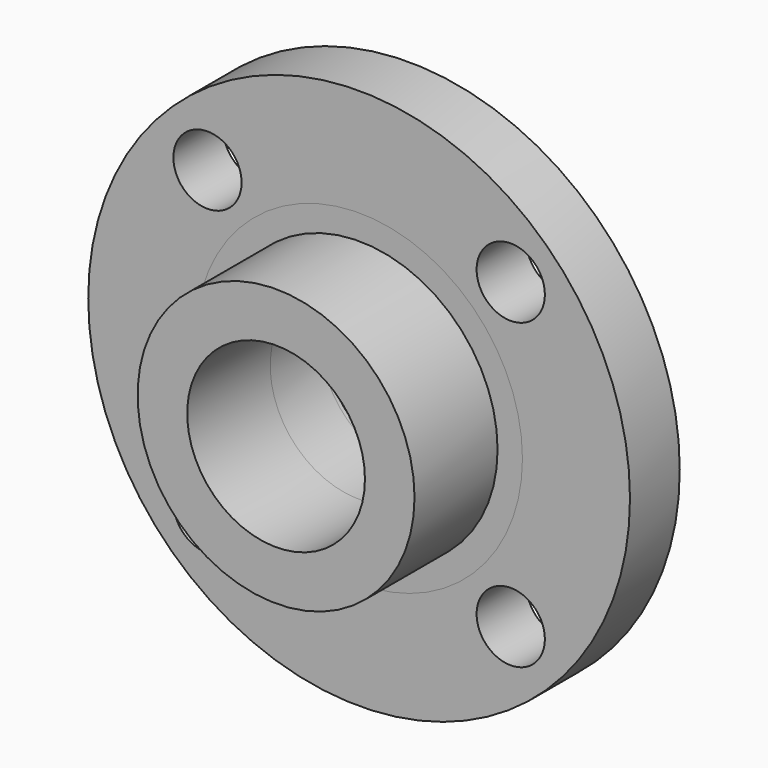
from build123d import *

# Parameters (mm, degrees)
F0_R     = 76.2
F0_R_2   = 9.6012
F0_R_3   = 9.595
F0_R_4   = 45.95
F1_DEPTH = 17.5
F0_R_5   = 25
F2_DEPTH = 1.14
F4_R     = 38.95
F4_R_2   = 25
F5_DEPTH = 29.2
F6_DEPTH = 17.5


# Not quite as in the source:
# - a fillet or chamfer that OpenCascade refuses, or shapes differently, is made with other operations: its cross-section is extruded or revolved along the edge and cut away or added


with BuildPart() as f1:
    # F0 (on Front) → F1 (new body)
    with BuildSketch(Plane.XZ):
        with Locations((-231.6003055891, 1.0374736618)):
            Circle(F0_R)
        with Locations((-274.2588413703, -41.6115579362)):
            Circle(F0_R_2, mode=Mode.SUBTRACT)
        with Locations((-188.9488413703, -41.6115579362)):
            Circle(F0_R_2, mode=Mode.SUBTRACT)
        with Locations((-274.2588413703, 43.6984420638)):
            Circle(F0_R_3, mode=Mode.SUBTRACT)
        with Locations((-231.6003055891, 1.0374736618)):
            Circle(F0_R_4, mode=Mode.SUBTRACT)
        with Locations((-188.9488413703, 43.6984420638)):
            Circle(F0_R_2, mode=Mode.SUBTRACT)
    extrude(amount=F1_DEPTH)


with BuildPart() as f2:
    # F0 (on Front) → F2 (new body)
    with BuildSketch(Plane.XZ):
        with Locations((-231.6003055891, 1.0374736618)):
            Circle(F0_R_4)
        with Locations((-231.6003055891, 1.0374736618)):
            Circle(F0_R_5, mode=Mode.SUBTRACT)
    extrude(amount=-F2_DEPTH)

    # F3: fillet of radius 5.08 on 1 edges, made by hand

    # F3_s1 → F3_t2 (revolve, cut)
    with BuildSketch(Plane.XY.offset(1.0374736618)):
        with BuildLine():
            ThreePointArc((-185.6503055891, 0), (-187.155339854, 0.8465227462), (-188.8569861157, 1.14))
            Line((-188.8569861157, 1.14), (-185.6503055891, 1.14))
            Line((-185.6503055891, 1.14), (-185.6503055891, 0))
        make_face()
    revolve(axis=Axis((-231.6003055891, 1.14, 1.0374736618), (0, -1, 0)), mode=Mode.SUBTRACT)


with BuildPart() as f5:
    # F4 (on face) → F5 (new body)
    with BuildSketch(Plane.XZ.offset(17.5)):
        with Locations((-231.6003055891, 1.0374736618)):
            Circle(F4_R)
        with Locations((-231.6003055891, 1.0374736618)):
            Circle(F4_R_2, mode=Mode.SUBTRACT)
    extrude(amount=F5_DEPTH)


with BuildPart() as f6:
    # F0 (on Front) → F6 (new body)
    with BuildSketch(Plane.XZ):
        with Locations((-231.6003055891, 1.0374736618)):
            Circle(F0_R_4)
        with Locations((-231.6003055891, 1.0374736618)):
            Circle(F0_R_5, mode=Mode.SUBTRACT)
    extrude(amount=F6_DEPTH)


solid = Compound([f1.part, f2.part, f5.part, f6.part])
